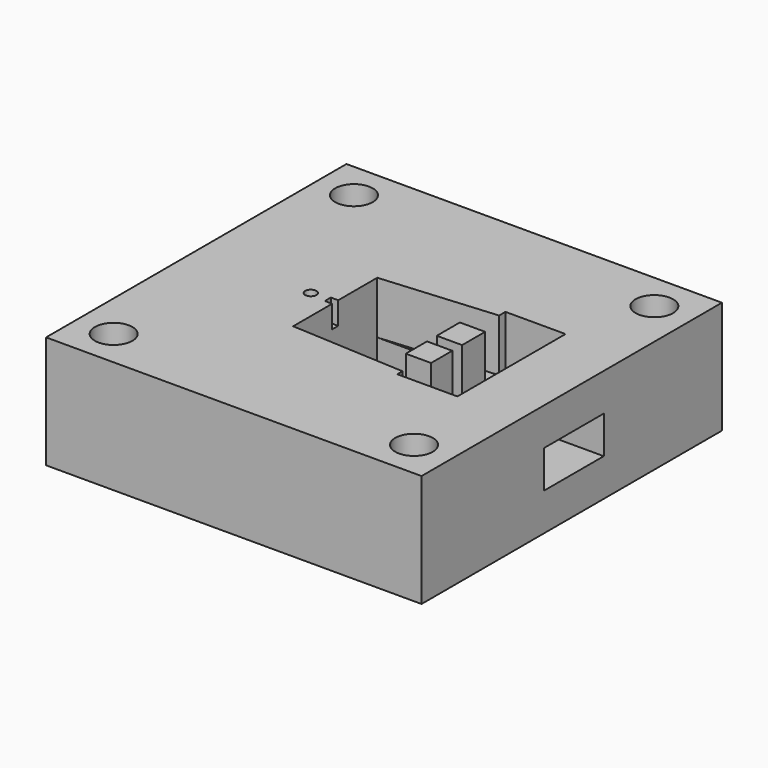
from build123d import *

# Parameters (mm, degrees)
F0_W           = 40
F0_H           = 40
F0_R           = 0.75
F0_W_2         = 13
F0_H_2         = 14
F1_DEPTH       = 10
F3_DEPTH       = 7
F5_DEPTH       = 7
F6_W           = 1
F6_H           = 10
F7_DEPTH       = 3
F9_W           = 40
F9_H           = 40
F9_W_2         = 13
F9_H_2         = 14
F10_DEPTH      = 5
F8_W           = 16.9138771733
F8_H           = 9.9888166223
F11_DEPTH      = 5
F13_W          = 3
F13_H          = 1.8063458446
F13_H_2        = 1.6774383839
F14_DEPTH      = 7
F15_W          = 50
F15_H          = 50
F15_W_2        = 40
F15_H_2        = 40
F16_DEPTH      = 10
F16_DEPTH_BACK = 5
F8_W_2         = 1
F8_W_3         = 4.5249774149
F8_W_4         = 11.3888997585
F18_DEPTH      = 5
F17_R          = 2.5
F19_DEPTH      = 15
F20_W          = 1
F20_H          = 18
F20_W_2        = 1.1054268107
F20_H_2        = 4.0429783403
F20_H_3        = 1.6282203142
F20_W_3        = 3.4427661449
F20_H_4        = 4.0144510567
F21_DEPTH      = 7
F22_W          = 1.9634229802
F22_H          = 1
F23_DEPTH      = 3


with BuildPart() as f1:
    # F0 (on Top) → F1 (new body)
    with BuildSketch(Plane.XY):
        with Locations((3.7967593362, -3.7976530202)):
            Rectangle(F0_W, F0_H)
        with Locations((-5.9532406638, -3.7976530202)):
            Circle(F0_R, mode=Mode.SUBTRACT)
        with Locations((3.7967593362, -3.7976530202)):
            Rectangle(F0_W_2, F0_H_2, mode=Mode.SUBTRACT)
    extrude(amount=F1_DEPTH)

    # F2 (on face) → F3 (cut)
    with BuildSketch(Plane.XY.offset(10)):
        Polygon((10.2967593362, -10.7976530202), (-2.7032406638, -10.7976530202), (19.3193775079, -11.9658830875), (19.2741411646, 5.0340567263), (-2.7032406638, 3.2023469798), (10.2967593362, 3.2023469798), (10.2967593362, -1.4381406363), (10.2967593362, -5.3588831797), align=None)
    extrude(amount=-F3_DEPTH, mode=Mode.SUBTRACT)

    # F4 (on face) → F5 (join)
    with BuildSketch(Plane.XY.offset(3)):
        Polygon((10.2967593362, -3.7976530202), (10.2967593362, -8.2976530202), (14.2967593362, -8.2976530202), (14.2967593362, 0.7023469798), (10.2967593362, 0.7023469798), align=None)
    extrude(amount=F5_DEPTH)

    # F6 (on face) → F7 (cut)
    with BuildSketch(Plane.XY.offset(3)):
        with Locations((18.7717819214, -3.4659131806)):
            Rectangle(F6_W, F6_H)
    extrude(amount=-F7_DEPTH, mode=Mode.SUBTRACT)

    # F9 (on face) → F10 (join)
    with BuildSketch(Plane(origin=(0, 0, 0), x_dir=(1, 0, 0), z_dir=(0, 0, -1))):
        with Locations((3.7967593362, 3.7976530202)):
            Rectangle(F9_W, F9_H)
        with Locations((3.7967593362, 3.7976530202)):
            Rectangle(F9_W_2, F9_H_2, mode=Mode.SUBTRACT)
    extrude(amount=F10_DEPTH)

    # F8 (on face) → F11 (cut)
    with BuildSketch(Plane(origin=(0, 0, 0), x_dir=(1, 0, 0), z_dir=(0, 0, -1))):
        with Locations((26.728720508, 3.4603214917)):
            Rectangle(F8_W, F8_H)
    extrude(amount=-F11_DEPTH, mode=Mode.SUBTRACT)

    # F13 (on face) → F14 (cut)
    with BuildSketch(Plane.XY.offset(10)):
        Polygon((19.5070204958, -12.4706726056), (19.5070204958, 5.5293273944), (15.5070204958, 5.5293273944), (15.5070204958, 3.7229815498), (15.5070204958, -10.7932342216), (15.5070204958, -12.4706726056), align=None)
        with Locations((14.0070204958, 4.6261544721)):
            Rectangle(F13_W, F13_H)
        with Locations((14.0070204958, -11.6319534136)):
            Rectangle(F13_W, F13_H_2)
    extrude(amount=-F14_DEPTH, mode=Mode.SUBTRACT)

    # F15 (on Top) → F16 (join, two sides)
    with BuildSketch(Plane.XY) as f16_sk:
        with Locations((3.7967593362, -3.7976530202)):
            Rectangle(F15_W, F15_H)
        with Locations((3.7967593362, -3.7976530202)):
            Rectangle(F15_W_2, F15_H_2, mode=Mode.SUBTRACT)
    extrude(amount=F16_DEPTH)
    extrude(f16_sk.sketch, amount=-F16_DEPTH_BACK)

    # F8 (on face) → F18 (cut)
    with BuildSketch(Plane(origin=(0, 0, 0), x_dir=(1, 0, 0), z_dir=(0, 0, -1))):
        with Locations((18.7717819214, 3.4603214917)):
            Rectangle(F8_W_2, F8_H)
        with Locations((21.5342706288, 3.4603214917)):
            Rectangle(F8_W_3, F8_H)
        with Locations((29.4912092155, 3.4603214917)):
            Rectangle(F8_W_4, F8_H)
    extrude(amount=-F18_DEPTH, mode=Mode.SUBTRACT)

    # F17 (on face) → F19 (cut)
    with BuildSketch(Plane.XY.offset(10)):
        with Locations((-16.2032406638, -23.7976530202)):
            Circle(F17_R)
        with Locations((-16.2032406638, 16.2023469798)):
            Circle(F17_R)
        with Locations((23.7967593362, -23.7976530202)):
            Circle(F17_R)
        with Locations((23.7967593362, 16.2023469798)):
            Circle(F17_R)
    extrude(amount=-F19_DEPTH, mode=Mode.SUBTRACT)

    # F20 (on face) → F21 (cut)
    with BuildSketch(Plane.XY.offset(10)):
        with Locations((20.0070204958, -3.4706726056)):
            Rectangle(F20_W, F20_H)
        with Locations((14.2178074457, -1.1141116556)):
            Rectangle(F20_W_2, F20_H_2)
        with Locations((14.2178074457, -3.9497109829)):
            Rectangle(F20_W_2, F20_H_3)
        with Locations((11.9437109679, -3.9497109829)):
            Rectangle(F20_W_3, F20_H_3)
        with Locations((14.2178074457, -6.7710466683)):
            Rectangle(F20_W_2, F20_H_4)
    extrude(amount=-F21_DEPTH, mode=Mode.SUBTRACT)

    # F22 (on face) → F23 (cut)
    with BuildSketch(Plane.XY.offset(10)):
        with Locations((-2.7032406638, -3.7976530202)):
            Rectangle(F22_W, F22_H)
    extrude(amount=-F23_DEPTH, mode=Mode.SUBTRACT)


solid = f1.part
